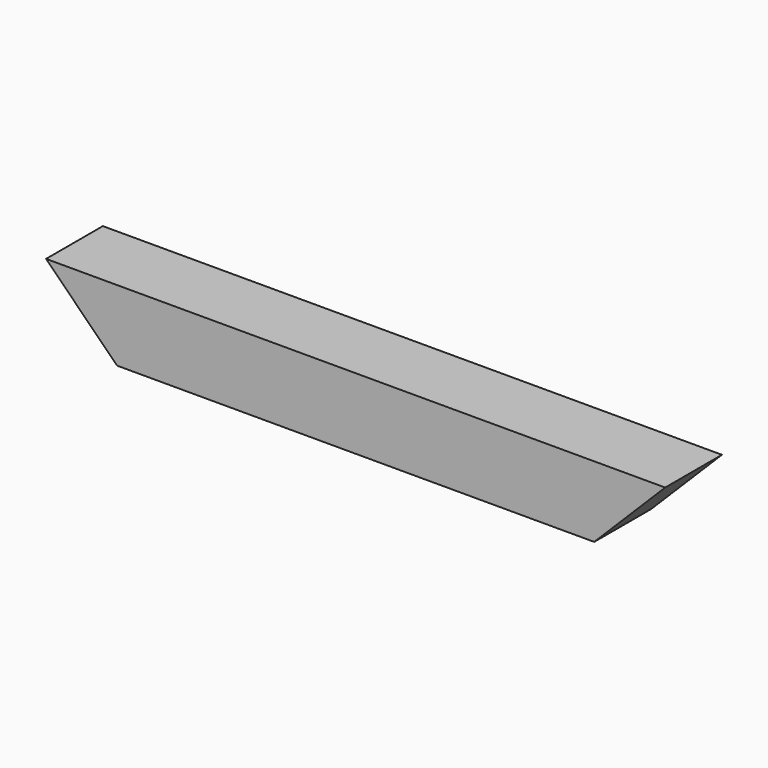
from build123d import *

# Parameters (mm, degrees)
F0_W     = 152.4
F0_H     = 17.4625
F1_DEPTH = 8.73125
F3_DEPTH = 17.4625
F4_DEPTH = 17.4625


# Not quite as in the source:
# - a length typed as a fraction of an inch, garbled in the dataset ("3 / 203.2 mm" for 3/8 in), is restored


with BuildPart() as f1:
    # F0 (on Front) → F1 (new body, symmetric)
    with BuildSketch(Plane.XZ):
        Rectangle(F0_W, F0_H)
    extrude(amount=F1_DEPTH, both=True)

    # F2 (on face) → F3 (cut)
    with BuildSketch(Plane.XZ.offset(8.73125)):
        Polygon((-58.7375, -8.73125), (-76.2, 8.73125), (-76.2, -8.73125), align=None)
    extrude(amount=-F3_DEPTH, mode=Mode.SUBTRACT)

    # F2 (on face) → F4 (cut)
    with BuildSketch(Plane.XZ.offset(8.73125)):
        Polygon((76.2, -8.73125), (76.2, 8.73125), (58.7375, -8.73125), align=None)
    extrude(amount=-F4_DEPTH, mode=Mode.SUBTRACT)


solid = f1.part
